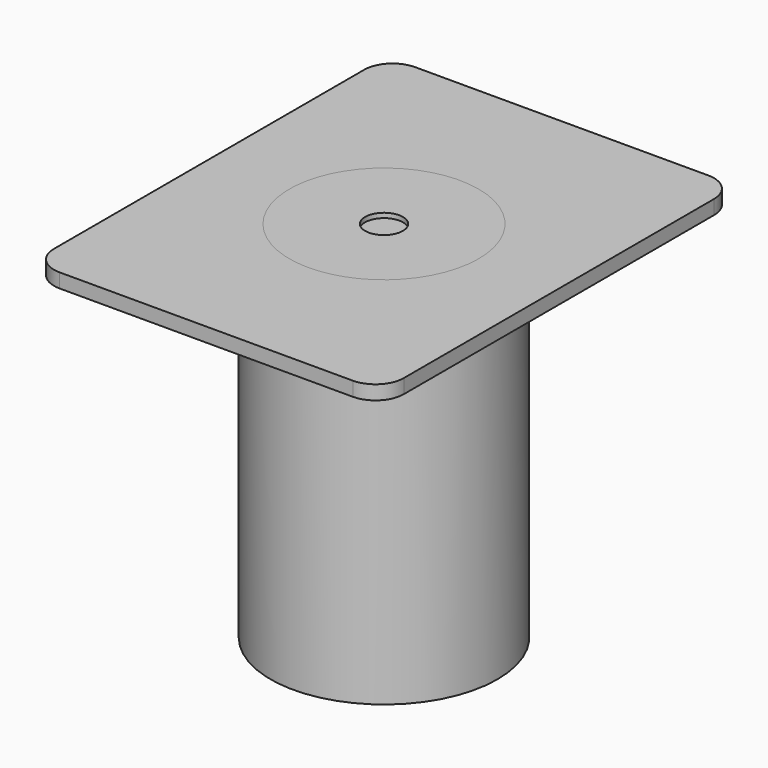
from build123d import *

# Parameters (mm, degrees)
F0_R      = 76.2
F1_DEPTH  = 234.95
F2_W      = 234.95
F2_H      = 298.45
F2_R      = 76.2
F3_DEPTH  = 9.525
F4_R      = 19.05
F6_DEPTH  = 3.175
F7_R      = 57.15
F8_DEPTH  = 241.301
F9_R      = 63.5
F9_R_2    = 12.7
F10_DEPTH = 3.175


# Not quite as in the source:
# - a length typed as a fraction of an inch, garbled in the dataset ("3 / 203.2 mm" for 3/8 in), is restored


with BuildPart() as f1:
    # F0 (on Top) → F1 (new body)
    with BuildSketch(Plane.XY):
        Circle(F0_R)
    extrude(amount=F1_DEPTH)


with BuildPart() as f3:
    # F2 (on face) → F3 (new body)
    with BuildSketch(Plane.XY.offset(234.95)):
        Rectangle(F2_W, F2_H)
        Circle(F2_R, mode=Mode.SUBTRACT)
        Circle(F2_R)
    extrude(amount=F3_DEPTH)

    # F4
    f4_edges = [f3.edges().sort_by_distance(p)[0] for p in [
        (117.475, -149.225, 239.7125),
        (-117.475, -149.225, 239.7125),
        (117.475, 149.225, 239.7125),
        (-117.475, 149.225, 239.7125),
    ]]
    fillet(f4_edges, radius=F4_R)

    # F5 (on face) → F6 (cut)
    with BuildSketch(Plane.XY.offset(244.475)):
        with BuildLine():
            ThreePointArc((-63.5, 0), (0, -63.5), (63.5, 0))
            Line((63.5, 0), (-63.5, 0))
        make_face()
        with BuildLine():
            Line((-63.5, 0), (63.5, 0))
            ThreePointArc((63.5, 0), (0, 63.5), (-63.5, 0))
        make_face()
    extrude(amount=-F6_DEPTH, mode=Mode.SUBTRACT)

    # F7 (on face) → F8 (cut, through all)
    with BuildSketch(Plane.XY.offset(241.3)):
        Circle(F7_R)
    extrude(amount=-F8_DEPTH, mode=Mode.SUBTRACT)


with BuildPart() as f10:
    # F9 (on face) → F10 (new body, through all)
    with BuildSketch(Plane.XY.offset(244.475)):
        Circle(F9_R)
        Circle(F9_R_2, mode=Mode.SUBTRACT)
    extrude(amount=-F10_DEPTH)


solid = Compound([f1.part, f3.part, f10.part])
